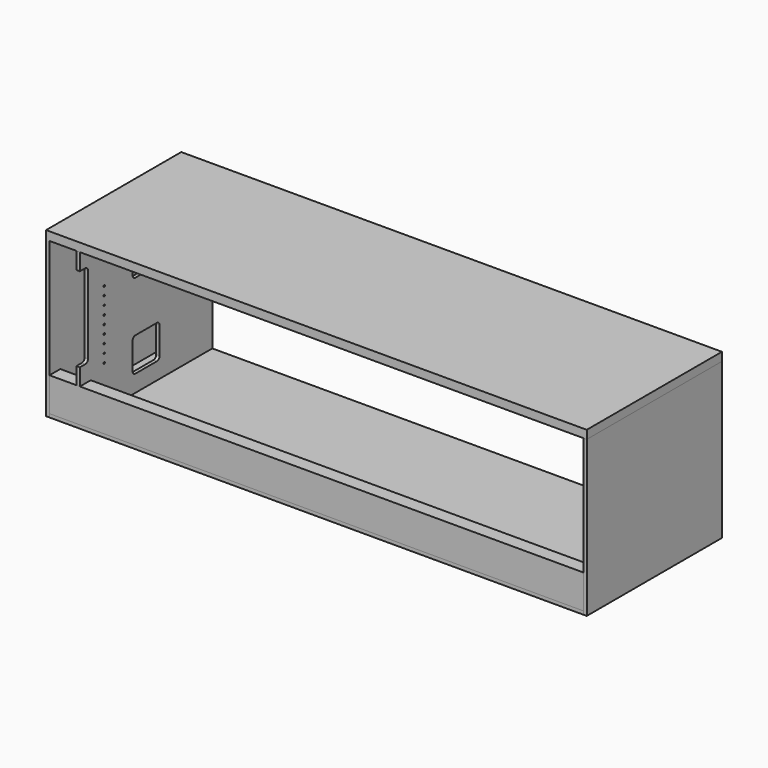
from build123d import *

# Parameters (mm, degrees)
F0_W      = 1600
F0_H      = 500
F1_DEPTH  = 25
F3_W      = 1580
F3_H      = 490
F4_DEPTH  = 10
F5_W      = 10
F5_H      = 500
F6_DEPTH  = 460
F7_W      = 10
F7_H      = 500
F8_DEPTH  = 460
F9_W      = 40
F9_H      = 100
F10_DEPTH = 1580
F11_W     = 10
F11_H     = 450
F12_DEPTH = 450
F13_W     = 10
F13_H     = 350
F14_DEPTH = 40
F16_W     = 30
F16_H     = 250
F17_DEPTH = 100.001
F18_R     = 10
F20_DEPTH = 100.001
F21_R     = 2.5
F22_DEPTH = 100.001


with BuildPart() as f1:
    # F0 (on Top) → F1 (new body)
    with BuildSketch(Plane.XY):
        with Locations((800, 250)):
            Rectangle(F0_W, F0_H)
    extrude(amount=F1_DEPTH)

    # F5 (on face) → F6 (join, through all)
    with BuildSketch(Plane.XY):
        with Locations((5, 250)):
            Rectangle(F5_W, F5_H)
    extrude(amount=-F6_DEPTH)


with BuildPart() as f4:
    # F3 (on offset) → F4 (new body)
    with BuildSketch(Plane.XY.offset(-460)):
        with Locations((800, 245)):
            Rectangle(F3_W, F3_H)
    extrude(amount=F4_DEPTH)


with BuildPart() as f8:
    # F7 (on face) → F8 (new body, through all)
    with BuildSketch(Plane.XY):
        with Locations((1595, 250)):
            Rectangle(F7_W, F7_H)
    extrude(amount=-F8_DEPTH)


with BuildPart() as f10:
    # F9 (on face) → F10 (new body, through all)
    with BuildSketch(Plane.YZ.offset(10)):
        with Locations((20, -400)):
            Rectangle(F9_W, F9_H)
    extrude(amount=F10_DEPTH)


with BuildPart() as f12:
    # F11 (on face) → F12 (new body, through all)
    with BuildSketch(Plane.XY.offset(-450)):
        with Locations((95, 265)):
            Rectangle(F11_W, F11_H)
    extrude(amount=F12_DEPTH)

    # F13 (on face) → F14 (join, through all)
    with BuildSketch(Plane.XZ.offset(-40)):
        with Locations((95, -175)):
            Rectangle(F13_W, F13_H)
    extrude(amount=F14_DEPTH)

    # F15: union 

    # F16 (on face) → F17 (cut, through all)
    with BuildSketch(Plane.YZ.offset(100)):
        with Locations((15, -175)):
            Rectangle(F16_W, F16_H)
    extrude(amount=-F17_DEPTH, mode=Mode.SUBTRACT)

    # F18
    f18_edges = [f12.edges().sort_by_distance(p)[0] for p in [
        (95, 30, -50),
        (95, 30, -300),
    ]]
    fillet(f18_edges, radius=F18_R)

    # F19 (on face) → F20 (cut, through all)
    with BuildSketch(Plane.YZ.offset(100)):
        with BuildLine():
            Line((285, -50), (205, -50))
            ThreePointArc((205, -50), (197.9289321881, -52.9289321881), (195, -60))
            Line((195, -60), (195, -140))
            ThreePointArc((195, -140), (197.9289321881, -147.0710678119), (205, -150))
            Line((205, -150), (285, -150))
            ThreePointArc((285, -150), (292.0710678119, -147.0710678119), (295, -140))
            Line((295, -140), (295, -60))
            ThreePointArc((295, -60), (292.0710678119, -52.9289321881), (285, -50))
        make_face()
        with BuildLine():
            Line((285, -300), (205, -300))
            ThreePointArc((205, -300), (197.9289321881, -302.9289321881), (195, -310))
            Line((195, -310), (195, -390))
            ThreePointArc((195, -390), (197.9289321881, -397.0710678119), (205, -400))
            Line((205, -400), (285, -400))
            ThreePointArc((285, -400), (292.0710678119, -397.0710678119), (295, -390))
            Line((295, -390), (295, -310))
            ThreePointArc((295, -310), (292.0710678119, -302.9289321881), (285, -300))
        make_face()
    extrude(amount=-F20_DEPTH, mode=Mode.SUBTRACT)

    # F21 (on face) → F22 (cut, through all)
    with BuildSketch(Plane.YZ.offset(100)):
        with Locations((90, -325)):
            Circle(F21_R)
        with Locations((90, -300)):
            Circle(F21_R)
        with Locations((90, -275)):
            Circle(F21_R)
        with Locations((90, -250)):
            Circle(F21_R)
        with Locations((90, -225)):
            Circle(F21_R)
        with Locations((90, -200)):
            Circle(F21_R)
        with Locations((90, -175)):
            Circle(F21_R)
        with Locations((90, -150)):
            Circle(F21_R)
        with Locations((90, -125)):
            Circle(F21_R)
    extrude(amount=-F22_DEPTH, mode=Mode.SUBTRACT)


solid = Compound([f1.part, f4.part, f8.part, f10.part, f12.part])
